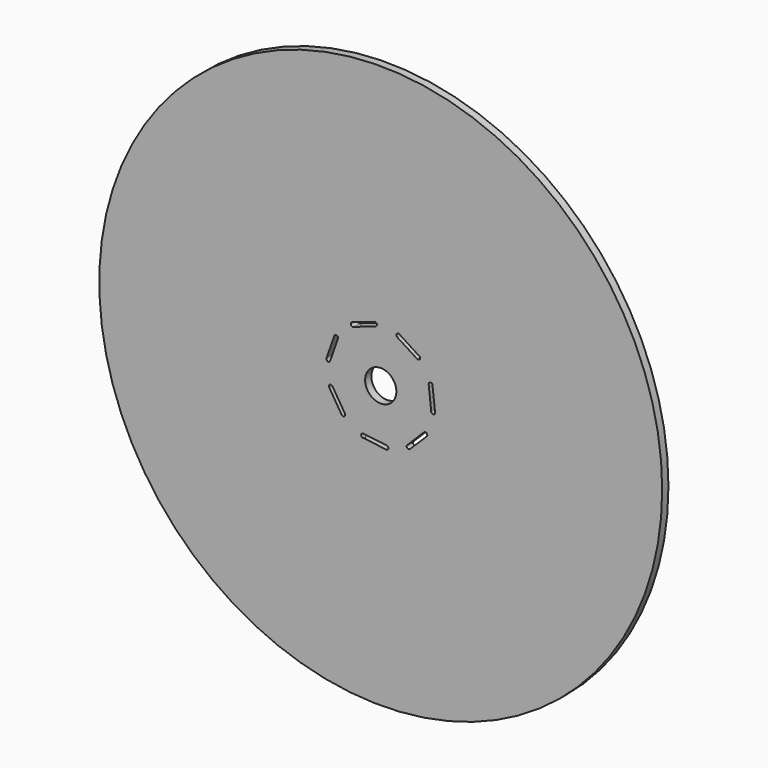
from build123d import *

# Parameters (mm, degrees)
F0_R     = 228.6
F1_DEPTH = 6.35
F3_DEPTH = 6.351
F4_R     = 12.7
F5_DEPTH = 6.351


# Not quite as in the source:
# - ends of sketch curves that miss each other by under 0.0002 mm in the source are joined


with BuildPart() as f1:
    # F0 (on Front) → F1 (new body)
    with BuildSketch(Plane.XZ):
        Circle(F0_R)
    extrude(amount=F1_DEPTH)

    # F2 (on face) → F3 (cut, through all)
    with BuildSketch(Plane(origin=(0, 0, 0), x_dir=(-1, 0, 0), z_dir=(0, 1, 0))):
        with BuildLine():
            Line((4.4618826202, 41.03312384), (22.1427530806, 34.8808349771))
            ThreePointArc((22.1427530806, 34.8808349771), (24.1653047772, 35.8628309135), (23.1774067066, 37.8825063297))
            Line((23.1774067066, 37.8825063297), (5.5701325615, 43.8941330325))
            Line((5.5701325615, 43.8941330325), (4.6801519701, 44.1979978468))
            ThreePointArc((4.6801519701, 44.1979978468), (3.5809145294, 43.7979774539), (3.0541190675, 42.7535519863))
            ThreePointArc((3.0541190675, 42.7535519863), (3.4066096848, 41.6058073542), (4.4618826202, 41.03312384))
        make_face()
        with BuildLine():
            Line((4.6801519701, 44.1979978468), (5.5701325615, 43.8941330325))
            ThreePointArc((5.5701325615, 43.8941330325), (5.1481595065, 44.1134796096), (4.6801519701, 44.1979978468))
        make_face()
        with BuildLine():
            Line((-31.727890274, 31.0981475896), (-30.7078696735, 31.753608073))
            ThreePointArc((-30.7078696735, 31.753608073), (-31.2829212175, 31.5270943199), (-31.727890274, 31.0981475896))
        make_face()
        with BuildLine():
            Line((-15.1702982711, 41.737979033), (-30.7078696735, 31.753608073))
            Line((-30.7078696735, 31.753608073), (-31.727890274, 31.0981475896))
            ThreePointArc((-31.727890274, 31.0981475896), (-31.5281772375, 29.050280341), (-29.4747442403, 28.9196721839))
            Line((-29.4747442403, 28.9196721839), (-13.4626581421, 39.061324038))
            ThreePointArc((-13.4626581421, 39.061324038), (-12.9781507091, 41.2534716), (-15.1702982711, 41.737979033))
        make_face()
        with BuildLine():
            Line((-40.992265014, -4.8302478058), (-38.9334293172, 13.8267433983))
            ThreePointArc((-38.9334293172, 13.8267433983), (-40.5597026781, 15.5876336173), (-42.0757424664, 13.7309907417))
            Line((-42.0757424664, 13.7309907417), (-44.151831017, -4.7859890094))
            ThreePointArc((-44.151831017, -4.7859890094), (-42.5964510469, -6.5502125075), (-40.992265014, -4.8302478058))
        make_face()
        with BuildLine():
            Line((34.8455227588, 22.1234679996), (41.0769142774, 4.4353792716))
            ThreePointArc((41.0769142774, 4.4353792716), (43.1041953835, 3.4664465633), (44.0697534768, 5.4953371086))
            Line((44.0697534768, 5.4953371086), (37.7754084063, 23.174174494))
            Line((37.7754084063, 23.174174494), (37.5676840132, 23.7576070393))
            ThreePointArc((37.5676840132, 23.7576070393), (35.3876634671, 24.3047338716), (34.8455227588, 22.1234679996))
        make_face()
        with BuildLine():
            Line((37.5676840132, 23.7576070393), (37.7754084063, 23.174174494))
            ThreePointArc((37.7754084063, 23.174174494), (37.7002728684, 23.4761185604), (37.5676840132, 23.7576070393))
        make_face()
        with BuildLine():
            Line((-23.6211183536, -37.6470325436), (-23.9224947466, -37.3484117712))
            ThreePointArc((-23.9224947466, -37.3484117712), (-23.7818274542, -37.5078355326), (-23.6211183536, -37.6470325436))
        make_face()
        with BuildLine():
            Line((-37.3220998756, -24.0713252866), (-23.9224947466, -37.3484117712))
            Line((-23.9224947466, -37.3484117712), (-23.6211183536, -37.6470325436))
            ThreePointArc((-23.6211183536, -37.6470325436), (-21.3089064889, -37.2063703199), (-21.9768545063, -34.9493031191))
            Line((-21.9768545063, -34.9493031191), (-35.0812263092, -21.8220953205))
            ThreePointArc((-35.0812263092, -21.8220953205), (-37.3262780755, -21.8262735204), (-37.3220998756, -24.0713252866))
        make_face()
        with BuildLine():
            Line((14.1274943747, -38.8257185152), (-4.6460917137, -41.0236705883))
            ThreePointArc((-4.6460917137, -41.0236705883), (-6.2226980939, -42.6185631758), (-4.6312320578, -44.1986283327))
            Line((-4.6312320578, -44.1986283327), (-4.2448360729, -44.1498861266))
            Line((-4.2448360729, -44.1498861266), (13.7359027682, -41.8816925861))
            Line((13.7359027682, -41.8816925861), (15.2375878216, -41.6922614193))
            ThreePointArc((15.2375878216, -41.6922614193), (15.7924641961, -39.8291626809), (14.1274943747, -38.8257185152))
        make_face()
        with BuildLine():
            Line((-4.2448360729, -44.1498861266), (-4.6312320578, -44.1986283327))
            ThreePointArc((-4.6312320578, -44.1986283327), (-4.4365336717, -44.1861513585), (-4.2448360729, -44.1498861266))
        make_face()
        with BuildLine():
            ThreePointArc((13.8057650277, -41.9070382349), (14.5475871245, -41.9723850949), (15.2375878216, -41.6922614193))
            Line((15.2375878216, -41.6922614193), (13.8057650277, -41.9070382349))
        make_face()
        with BuildLine():
            Line((13.8057650277, -41.9070382349), (15.2375878216, -41.6922614193))
            Line((15.2375878216, -41.6922614193), (13.7359027682, -41.8816925861))
            ThreePointArc((13.7359027682, -41.8816925861), (13.7706855601, -41.8947742862), (13.8057650277, -41.9070382349))
        make_face()
        with BuildLine():
            Line((39.1205111726, -13.2355457292), (29.0774053416, -29.3519750753))
            ThreePointArc((29.0774053416, -29.3519750753), (29.5860528198, -31.5394518473), (31.7731794636, -31.0293009591))
            Line((31.7731794636, -31.0293009591), (41.6947378015, -15.0590532006))
            Line((41.6947378015, -15.0590532006), (41.9843072327, -14.5929474337))
            ThreePointArc((41.9843072327, -14.5929474337), (41.1912924211, -12.5663543268), (39.1205111726, -13.2355457292))
        make_face()
        with BuildLine():
            Line((41.9843072327, -14.5929474337), (41.6947378015, -15.0590532006))
            ThreePointArc((41.6947378015, -15.0590532006), (41.8598142795, -14.8386066278), (41.9843072327, -14.5929474337))
        make_face()
    extrude(amount=-F3_DEPTH, mode=Mode.SUBTRACT)

    # F4 (on face) → F5 (cut, through all)
    with BuildSketch(Plane.XZ.offset(6.35)):
        Circle(F4_R)
    extrude(amount=-F5_DEPTH, mode=Mode.SUBTRACT)


solid = f1.part
